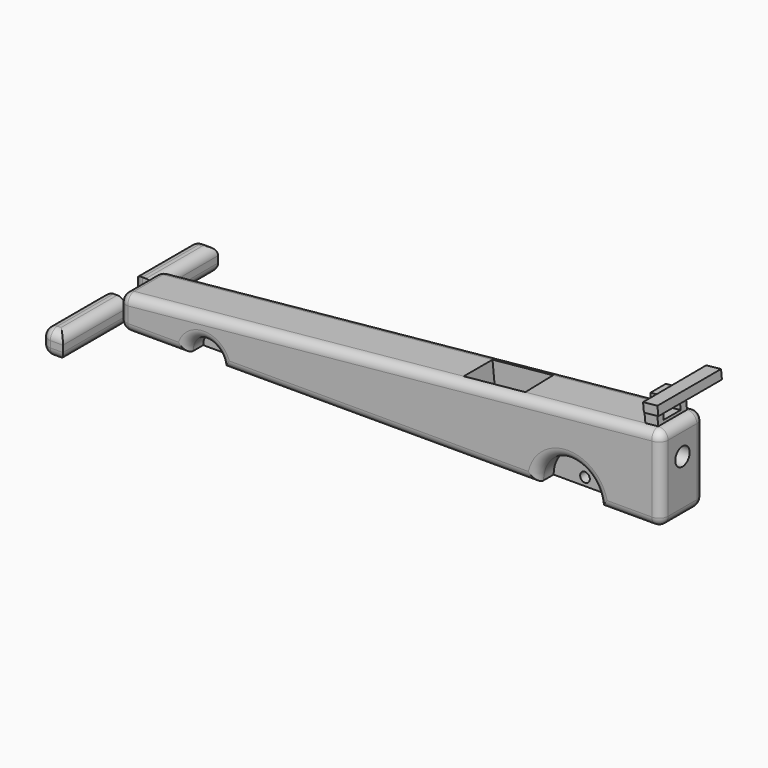
from build123d import *

# Parameters (mm, degrees)
F1_DEPTH        = 30
F2_R            = 10
F2_R_2          = 17.5
F3_DEPTH        = 12
F4_R            = 10
F4_R_2          = 17.5
F5_DEPTH        = 12
F6_R            = 5
F7_W            = 7.1860023443
F7_H            = 20
F8_DEPTH        = 10
F10_DEPTH       = 2.5
F12_DEPTH       = 5
F13_W           = 11.7590613663
F13_H           = 5.7444307604
F14_DEPTH       = 25
F15_R           = 2.0212258773
F16_DEPTH       = 25
F17_R           = 2.6949669584
F18_DEPTH       = 25
F19_W           = 44
F19_H           = 13.599084351
F20_DEPTH       = 12
F21_T1_DEPTH    = 20
F21_S5_W        = 5
F21_S5_H        = 5
F21_T6_DEPTH    = 5
F21_S11_W       = 5
F21_S11_H       = 5
F21_T12_DEPTH   = 5
F21_2_T1_DEPTH  = 51.5
F21_2_T3_DEPTH  = 34
F21_2_T5_DEPTH  = 3.599084351
F21_2_T7_DEPTH  = 21.099084351
F21_2_T9_DEPTH  = 19.5
F21_2_T11_DEPTH = 69
F21_2_S15_W     = 5
F21_2_S15_H     = 5
F21_2_T16_DEPTH = 5
F21_2_S21_W     = 5
F21_2_S21_H     = 5
F21_2_T22_DEPTH = 5
F21_2_S27_W     = 5
F21_2_S27_H     = 5
F21_2_T28_DEPTH = 5
F21_3_T1_DEPTH  = 51.5
F21_3_T3_DEPTH  = 3.5990095853
F21_3_T5_DEPTH  = 34.0000000001
F21_3_T7_DEPTH  = 19.4999760367
F21_3_T9_DEPTH  = 19.5
F21_3_T11_DEPTH = 21.0990747656
F21_3_T13_DEPTH = 69.0000000001
F21_3_T15_DEPTH = 19.5000239634
F21_3_T17_DEPTH = 69
F21_3_S21_W     = 5
F21_3_S21_H     = 5
F21_3_T22_DEPTH = 5
F21_3_T28_DEPTH = 5
F21_3_T34_DEPTH = 5
F23_DEPTH       = 15
F24_R           = 5
F25_DEPTH       = 10


# Not quite as in the source:
# - a fillet or chamfer that OpenCascade refuses, or shapes differently, is made with other operations: its cross-section is extruded or revolved along the edge and cut away or added


with BuildPart() as f1:
    # F0 (on Front) → F1 (new body)
    with BuildSketch(Plane.XZ):
        Polygon((-158.1492722034, -17.9878585041), (-158.1492722034, -36.1196212471), (143.4711813927, -36.1196212471), (143.4711813927, 11.656133458), align=None)
    extrude(amount=F1_DEPTH)

    # F2 (on face) → F3 (cut)
    with BuildSketch(Plane.XZ.offset(30)):
        with Locations((-110.8754724264, -36.1196212471)):
            Circle(F2_R)
        with Locations((91.665007174, -36.1196212471)):
            Circle(F2_R_2)
    extrude(amount=-F3_DEPTH, mode=Mode.SUBTRACT)

    # F4 (on face) → F5 (cut)
    with BuildSketch(Plane(origin=(0, 0, 0), x_dir=(-1, 0, 0), z_dir=(0, 1, 0))):
        with Locations((109.850294888, -36.1196212471)):
            Circle(F4_R)
        with Locations((-90.4239937663, -36.1196212471)):
            Circle(F4_R_2)
    extrude(amount=-F5_DEPTH, mode=Mode.SUBTRACT)

    # F6
    f6_edges = [f1.edges().sort_by_distance(p)[0] for p in [
        (-158.149272, -15, -17.987859),
        (-7.339045, -30, -3.165863),
        (-110.875472, -30, -26.119621),
        (-158.149272, -30, -27.05374),
        (91.665007, -30, -18.619621),
        (-158.149272, 0, -27.05374),
        (-109.850295, 0, -26.119621),
        (90.423994, 0, -18.619621),
        (-7.339045, 0, -3.165863),
        (143.471181, 0, -12.231744),
        (143.471181, -30, -12.231744),
        (143.471181, -15, 11.656133),
        (-13.463151, 0, -36.119621),
        (-13.355233, -30, -36.119621),
        (126.318094, -30, -36.119621),
        (125.697588, 0, -36.119621),
        (-138.999784, 0, -36.119621),
        (-139.512372, -30, -36.119621),
        (143.471181, -15, -36.119621),
    ]]
    fillet(f6_edges, radius=F6_R)

    # F7 (on face) → F8 (join)
    with BuildSketch(Plane(origin=(0.2379590763, 0, -2.4211760892), x_dir=(0.9952049917, 0, 0.0978111677), z_dir=(-0.0978111677, 0, 0.9952049917))):
        with Locations((134.814832017, -15)):
            Rectangle(F7_W, F7_H)
    extrude(amount=F8_DEPTH)

    # F9 (on face) → F10 (join)
    with BuildSketch(Plane(origin=(-0.7401526009, 0, 7.5308738276), x_dir=(0.9952049917, 0, 0.0978111677), z_dir=(-0.0978111677, 0, 0.9952049917))):
        Polygon((145.5644071102, -9.13162902), (131.2218308449, -9.2158466578), (131.2218308449, -19.9957098812), (145.5644071102, -19.9957098812), align=None)
    extrude(amount=F10_DEPTH)

    # F11 (on face) → F12 (join)
    with BuildSketch(Plane(origin=(-0.9846805202, 0, 10.0188863068), x_dir=(0.9952049917, 0, 0.0978111677), z_dir=(-0.0978111677, 0, 0.9952049917))):
        Polygon((150.0439193667, 6.3689760585), (141.7933106422, 6.3205296174), (142.0532540115, -37.9487908802), (150.0439193667, -37.8912001254), align=None)
    extrude(amount=F12_DEPTH)

    # F13 (on face) → F14 (cut)
    with BuildSketch(Plane(origin=(130.5926210745, 0, 12.8349605051), x_dir=(0, -1, 0), z_dir=(-0.9952049917, 0, -0.0978111677))):
        with Locations((15.0953773409, 1.9727416511)):
            Rectangle(F13_W, F13_H)
    extrude(amount=-F14_DEPTH, mode=Mode.SUBTRACT)

    # F15 (on face) → F16 (cut)
    with BuildSketch(Plane.XZ.offset(18)):
        with Locations((-111.3435998559, -32.4539355934)):
            Circle(F15_R)
    extrude(amount=-F16_DEPTH, mode=Mode.SUBTRACT)

    # F17 (on face) → F18 (cut)
    with BuildSketch(Plane.XZ.offset(18)):
        with Locations((91.6058570147, -31.7393243313)):
            Circle(F17_R)
    extrude(amount=-F18_DEPTH, mode=Mode.SUBTRACT)

    # F21: fillet of radius 5 on 1 edges, made by hand

    # F21_s2 → F21_t1 (cut)
    with BuildSketch(Plane.XZ.offset(5)):
        with BuildLine():
            ThreePointArc((-158.1492722034, -31.1196212471), (-156.6848061094, -34.655155153), (-153.1492722034, -36.1196212471))
            Line((-153.1492722034, -36.1196212471), (-158.1492722034, -36.1196212471))
            Line((-158.1492722034, -36.1196212471), (-158.1492722034, -31.1196212471))
        make_face()
    extrude(amount=F21_T1_DEPTH, mode=Mode.SUBTRACT)


with BuildPart() as f20:
    # F19 (on face) → F20 (new body)
    with BuildSketch(Plane(origin=(-158.1492722034, 0, 0), x_dir=(0, -1, 0), z_dir=(-1, 0, 0))):
        with Locations((-17, -29.3200790716)):
            Rectangle(F19_W, F19_H)
    extrude(amount=F20_DEPTH)

    # F21#2: fillet of radius 5 on 9 edges, made by hand

    # F21_2_s2 → F21_2_t1 (cut)
    with BuildSketch(Plane.XZ.offset(-34)):
        with BuildLine():
            ThreePointArc((-165.1492722034, -22.5205368961), (-168.6848061094, -23.9850029901), (-170.1492722034, -27.5205368961))
            Line((-170.1492722034, -27.5205368961), (-170.1492722034, -22.5205368961))
            Line((-170.1492722034, -22.5205368961), (-165.1492722034, -22.5205368961))
        make_face()
    extrude(amount=F21_2_T1_DEPTH, mode=Mode.SUBTRACT)

    # F21_2_s4 → F21_2_t3 (cut)
    with BuildSketch(Plane.XZ.offset(-34)):
        with BuildLine():
            ThreePointArc((-165.1492722034, -36.1196212471), (-168.6848061094, -34.655155153), (-170.1492722034, -31.1196212471))
            Line((-170.1492722034, -31.1196212471), (-170.1492722034, -36.1196212471))
            Line((-170.1492722034, -36.1196212471), (-165.1492722034, -36.1196212471))
        make_face()
    extrude(amount=F21_2_T3_DEPTH, mode=Mode.SUBTRACT)

    # F21_2_s6 → F21_2_t5 (cut)
    with BuildSketch(Plane.XY.offset(-31.1196212471)):
        with BuildLine():
            ThreePointArc((-165.1492722034, 39), (-168.6848061094, 37.5355339059), (-170.1492722034, 34))
            Line((-170.1492722034, 34), (-170.1492722034, 39))
            Line((-170.1492722034, 39), (-165.1492722034, 39))
        make_face()
    extrude(amount=F21_2_T5_DEPTH, mode=Mode.SUBTRACT)

    # F21_2_s8 → F21_2_t7 (cut)
    with BuildSketch(Plane.XY.offset(-31.1196212471)):
        with BuildLine():
            ThreePointArc((-165.1492722034, -5), (-168.6848061094, -3.5355339059), (-170.1492722034, 0))
            Line((-170.1492722034, 0), (-170.1492722034, -5))
            Line((-170.1492722034, -5), (-165.1492722034, -5))
        make_face()
    extrude(amount=F21_2_T7_DEPTH, mode=Mode.SUBTRACT)

    # F21_2_s10 → F21_2_t9 (cut)
    with BuildSketch(Plane.YZ.offset(-165.1492722034)):
        with BuildLine():
            ThreePointArc((34, -22.5205368961), (37.5355339059, -23.9850029901), (39, -27.5205368961))
            Line((39, -27.5205368961), (39, -22.5205368961))
            Line((39, -22.5205368961), (34, -22.5205368961))
        make_face()
        with BuildLine():
            ThreePointArc((39, -31.1196212471), (37.5355339059, -34.655155153), (34, -36.1196212471))
            Line((34, -36.1196212471), (39, -36.1196212471))
            Line((39, -36.1196212471), (39, -31.1196212471))
        make_face()
        with BuildLine():
            ThreePointArc((-5, -31.1196212471), (-3.5355339059, -34.655155153), (0, -36.1196212471))
            Line((0, -36.1196212471), (-5, -36.1196212471))
            Line((-5, -36.1196212471), (-5, -31.1196212471))
        make_face()
    extrude(amount=F21_2_T9_DEPTH, mode=Mode.SUBTRACT)

    # F21_2_s12 → F21_2_t11 (cut)
    with BuildSketch(Plane.XZ.offset(-51.5)):
        with BuildLine():
            ThreePointArc((-163.1492722034, -36.1196212471), (-159.6137382975, -34.655155153), (-158.1492722034, -31.1196212471))
            Line((-158.1492722034, -31.1196212471), (-158.1492722034, -36.1196212471))
            Line((-158.1492722034, -36.1196212471), (-163.1492722034, -36.1196212471))
        make_face()
        with BuildLine():
            ThreePointArc((-163.1492722034, -22.5205368961), (-159.6137382975, -23.9850029901), (-158.1492722034, -27.5205368961))
            Line((-158.1492722034, -27.5205368961), (-158.1492722034, -22.5205368961))
            Line((-158.1492722034, -22.5205368961), (-163.1492722034, -22.5205368961))
        make_face()
    extrude(amount=F21_2_T11_DEPTH, mode=Mode.SUBTRACT)


with BuildPart() as f20b:
    # F19 (on face) → F20, piece 2 (new body)
    with BuildSketch(Plane(origin=(-158.1492722034, 0, 0), x_dir=(0, -1, 0), z_dir=(-1, 0, 0))):
        Polygon((69, -22.5205368961), (25, -22.5205368961), (25, -36.1196212471), (69, -36.1195368961), align=None)
    extrude(amount=F20_DEPTH)

    # F21#3: fillet of radius 5 on 9 edges, made by hand

    # F21_3_s2 → F21_3_t1 (cut)
    with BuildSketch(Plane.XZ.offset(12.5)):
        with BuildLine():
            ThreePointArc((-165.1492722034, -22.5205368961), (-168.6848061094, -23.9850029901), (-170.1492722034, -27.5205368961))
            Line((-170.1492722034, -27.5205368961), (-170.1492722034, -22.5205368961))
            Line((-170.1492722034, -22.5205368961), (-165.1492722034, -22.5205368961))
        make_face()
    extrude(amount=F21_3_T1_DEPTH, mode=Mode.SUBTRACT)

    # F21_3_s4 → F21_3_t3 (cut)
    with BuildSketch(Plane.XY.offset(-31.1195464814)):
        with BuildLine():
            ThreePointArc((-165.1492722034, -69), (-168.6848061094, -67.5355339059), (-170.1492722034, -64))
            Line((-170.1492722034, -64), (-170.1492722034, -69))
            Line((-170.1492722034, -69), (-165.1492722034, -69))
        make_face()
    extrude(amount=F21_3_T3_DEPTH, mode=Mode.SUBTRACT)

    # F21_3_s6 → F21_3_t5 (cut)
    with BuildSketch(Plane(origin=(0, -29.9999403415, 5.75119e-05), x_dir=(1, 0, 0), z_dir=(0, -1, 1.9171e-06))):
        with BuildLine():
            ThreePointArc((-165.1492722034, -36.1196691737), (-168.6848061094, -34.6552030796), (-170.1492722034, -31.1196691737))
            Line((-170.1492722034, -31.1196691737), (-170.1492722034, -36.1196691737))
            Line((-170.1492722034, -36.1196691737), (-165.1492722034, -36.1196691737))
        make_face()
    extrude(amount=F21_3_T5_DEPTH, mode=Mode.SUBTRACT)

    # F21_3_s8 → F21_3_t7 (cut)
    with BuildSketch(Plane.YZ.offset(-165.1492722034)):
        with BuildLine():
            ThreePointArc((-69, -31.1195464814), (-67.5355372949, -34.6550769984), (-64.0000095853, -36.1195464814))
            Line((-64.0000095853, -36.1195464814), (-69, -36.1195368961))
            Line((-69, -36.1195368961), (-69, -31.1195464814))
        make_face()
    extrude(amount=F21_3_T7_DEPTH, mode=Mode.SUBTRACT)

    # F21_3_s10 → F21_3_t9 (cut)
    with BuildSketch(Plane.YZ.offset(-165.1492722034)):
        with BuildLine():
            ThreePointArc((-69, -27.5205368961), (-67.5355339059, -23.9850029901), (-64, -22.5205368961))
            Line((-64, -22.5205368961), (-69, -22.5205368961))
            Line((-69, -22.5205368961), (-69, -27.5205368961))
        make_face()
    extrude(amount=F21_3_T9_DEPTH, mode=Mode.SUBTRACT)

    # F21_3_s12 → F21_3_t11 (cut)
    with BuildSketch(Plane.XY.offset(-31.1196116617)):
        with BuildLine():
            ThreePointArc((-165.1492722034, -25), (-168.6848061094, -26.4644660941), (-170.1492722034, -30))
            Line((-170.1492722034, -30), (-170.1492722034, -25))
            Line((-170.1492722034, -25), (-165.1492722034, -25))
        make_face()
    extrude(amount=F21_3_T11_DEPTH, mode=Mode.SUBTRACT)

    # F21_3_s14 → F21_3_t13 (cut)
    with BuildSketch(Plane(origin=(0, -12.4999307562, 2.39632e-05), x_dir=(1, 0, 0), z_dir=(0, -1, 1.9171e-06))):
        with BuildLine():
            ThreePointArc((-163.1492722034, -36.1196691737), (-159.6137382975, -34.6552030796), (-158.1492722034, -31.1196691737))
            Line((-158.1492722034, -31.1196691737), (-158.1492722034, -36.1196691737))
            Line((-158.1492722034, -36.1196691737), (-163.1492722034, -36.1196691737))
        make_face()
    extrude(amount=F21_3_T13_DEPTH, mode=Mode.SUBTRACT)

    # F21_3_s16 → F21_3_t15 (cut)
    with BuildSketch(Plane.YZ.offset(-165.1492722034)):
        with BuildLine():
            ThreePointArc((-25, -31.1196116617), (-26.464469483, -34.6551489566), (-30.0000095853, -36.1196116617))
            Line((-30.0000095853, -36.1196116617), (-25, -36.1196212471))
            Line((-25, -36.1196212471), (-25, -31.1196116617))
        make_face()
    extrude(amount=F21_3_T15_DEPTH, mode=Mode.SUBTRACT)

    # F21_3_s18 → F21_3_t17 (cut)
    with BuildSketch(Plane.XZ.offset(12.5)):
        with BuildLine():
            ThreePointArc((-163.1492722034, -22.5205368961), (-159.6137382975, -23.9850029901), (-158.1492722034, -27.5205368961))
            Line((-158.1492722034, -27.5205368961), (-158.1492722034, -22.5205368961))
            Line((-158.1492722034, -22.5205368961), (-163.1492722034, -22.5205368961))
        make_face()
    extrude(amount=F21_3_T17_DEPTH, mode=Mode.SUBTRACT)


with BuildPart() as f21_tool4:
    # F21_s5 → F21_t6 (new body)
    with BuildSketch(Plane.YZ.offset(-153.1492722034)):
        with Locations((-2.5, -33.6196212471)):
            Rectangle(F21_S5_W, F21_S5_H)
    extrude(amount=-F21_T6_DEPTH)

    # F21_s7 → F21_t8 (revolve, cut)
    with BuildSketch(Plane(origin=(-153.1492722034, -5, -31.1196212471), x_dir=(0, -0.7071067812, 0.7071067812), z_dir=(0, -0.7071067812, -0.7071067812))):
        with BuildLine():
            ThreePointArc((0, -5), (5, 0), (0, 5))
            Line((0, 5), (0, -5))
        make_face()
    revolve(axis=Axis((-153.1492722034, -5, -31.1196212471), (-1, 0, 0)), mode=Mode.SUBTRACT)


with BuildPart() as f1_1:
    add(f1.part)

    # F21_t3: cut F21_tool4
    add(f21_tool4.part, mode=Mode.SUBTRACT)


with BuildPart() as f21_tool10:
    # F21_s11 → F21_t12 (new body)
    with BuildSketch(Plane.YZ.offset(-153.1492722034)):
        with Locations((-27.5, -33.6196212471)):
            Rectangle(F21_S11_W, F21_S11_H)
    extrude(amount=-F21_T12_DEPTH)

    # F21_s13 → F21_t14 (revolve, cut)
    with BuildSketch(Plane(origin=(-153.1492722034, -25, -31.1196212471), x_dir=(0, 0.7071067812, 0.7071067812), z_dir=(0, -0.7071067812, 0.7071067812))):
        with BuildLine():
            ThreePointArc((0, -5), (5, 0), (0, 5))
            Line((0, 5), (0, -5))
        make_face()
    revolve(axis=Axis((-153.1492722034, -25, -31.1196212471), (-1, 0, 0)), mode=Mode.SUBTRACT)


with BuildPart() as f1_2:
    add(f1_1.part)

    # F21_t9: cut F21_tool10
    add(f21_tool10.part, mode=Mode.SUBTRACT)

    # F22 (on face) → F23 (cut)
    with BuildSketch(Plane(origin=(0.2379590763, 0, -2.4211760892), x_dir=(0.9952049917, 0, 0.0978111677), z_dir=(-0.0978111677, 0, 0.9952049917))):
        Polygon((64.090423286, -25), (63.5211393237, -5), (29.6491980553, -5), (29.6491980553, -25), align=None)
    extrude(amount=-F23_DEPTH, mode=Mode.SUBTRACT)

    # F24 (on face) → F25 (cut)
    with BuildSketch(Plane.YZ.offset(143.4711813927)):
        with Locations((-15, -5.9098936617)):
            Circle(F24_R)
    extrude(amount=-F25_DEPTH, mode=Mode.SUBTRACT)


with BuildPart() as f21_2_tool14:
    # F21_2_s15 → F21_2_t16 (new body)
    with BuildSketch(Plane.XY.offset(-27.5205368961)):
        with Locations((-167.6492722034, 36.5)):
            Rectangle(F21_2_S15_W, F21_2_S15_H)
    extrude(amount=F21_2_T16_DEPTH)

    # F21_2_s17 → F21_2_t18 (revolve, cut)
    with BuildSketch(Plane(origin=(-165.1492722034, 34, -27.5205368961), x_dir=(0.7071067812, -0.7071067812, 0), z_dir=(-0.7071067812, -0.7071067812, 0))):
        with BuildLine():
            ThreePointArc((0, -5), (5, 0), (0, 5))
            Line((0, 5), (0, -5))
        make_face()
    revolve(axis=Axis((-165.1492722034, 34, -27.5205368961), (0, 0, 1)), mode=Mode.SUBTRACT)


with BuildPart() as f20_1:
    add(f20.part)

    # F21_2_t13: cut F21_2_tool14
    add(f21_2_tool14.part, mode=Mode.SUBTRACT)


with BuildPart() as f21_2_tool20:
    # F21_2_s21 → F21_2_t22 (new body)
    with BuildSketch(Plane.XZ.offset(-34)):
        with Locations((-167.6492722034, -33.6196212471)):
            Rectangle(F21_2_S21_W, F21_2_S21_H)
    extrude(amount=-F21_2_T22_DEPTH)

    # F21_2_s23 → F21_2_t24 (revolve, cut)
    with BuildSketch(Plane(origin=(-165.1492722034, 34, -31.1196212471), x_dir=(0.7071067812, 0, 0.7071067812), z_dir=(-0.7071067812, 0, 0.7071067812))):
        with BuildLine():
            ThreePointArc((0, -5), (5, 0), (0, 5))
            Line((0, 5), (0, -5))
        make_face()
    revolve(axis=Axis((-165.1492722034, 34, -31.1196212471), (0, 1, 0)), mode=Mode.SUBTRACT)


with BuildPart() as f20_2:
    add(f20_1.part)

    # F21_2_t19: cut F21_2_tool20
    add(f21_2_tool20.part, mode=Mode.SUBTRACT)


with BuildPart() as f21_2_tool26:
    # F21_2_s27 → F21_2_t28 (new body)
    with BuildSketch(Plane.XZ):
        with Locations((-167.6492722034, -33.6196212471)):
            Rectangle(F21_2_S27_W, F21_2_S27_H)
    extrude(amount=F21_2_T28_DEPTH)

    # F21_2_s29 → F21_2_t30 (revolve, cut)
    with BuildSketch(Plane(origin=(-165.1492722034, 0, -31.1196212471), x_dir=(0.7071067812, 0, 0.7071067812), z_dir=(0.7071067812, 0, -0.7071067812))):
        with BuildLine():
            ThreePointArc((0, -5), (5, 0), (0, 5))
            Line((0, 5), (0, -5))
        make_face()
    revolve(axis=Axis((-165.1492722034, 0, -31.1196212471), (0, -1, 0)), mode=Mode.SUBTRACT)


with BuildPart() as f20_3:
    add(f20_2.part)

    # F21_2_t25: cut F21_2_tool26
    add(f21_2_tool26.part, mode=Mode.SUBTRACT)


with BuildPart() as f21_3_tool20:
    # F21_3_s21 → F21_3_t22 (new body)
    with BuildSketch(Plane.XZ.offset(64)):
        with Locations((-167.6492722034, -25.0205368961)):
            Rectangle(F21_3_S21_W, F21_3_S21_H)
    extrude(amount=F21_3_T22_DEPTH)

    # F21_3_s23 → F21_3_t24 (revolve, cut)
    with BuildSketch(Plane(origin=(-165.1492722034, -64, -27.5205368961), x_dir=(0.7071067812, 0, -0.7071067812), z_dir=(-0.7071067812, 0, -0.7071067812))):
        with BuildLine():
            ThreePointArc((0, -5), (5, 0), (0, 5))
            Line((0, 5), (0, -5))
        make_face()
    revolve(axis=Axis((-165.1492722034, -64, -27.5205368961), (0, -1, 0)), mode=Mode.SUBTRACT)


with BuildPart() as f20b_1:
    add(f20b.part)

    # F21_3_t19: cut F21_3_tool20
    add(f21_3_tool20.part, mode=Mode.SUBTRACT)


with BuildPart() as f21_3_tool26:
    # F21_3_s27 → F21_3_t28 (new body)
    with BuildSketch(Plane.YZ.offset(-165.1492722034)):
        Polygon((-64, -31.1195464814), (-69, -31.1195464814), (-69, -36.1195368961), (-64.0000095853, -36.1195464814), align=None)
    extrude(amount=-F21_3_T28_DEPTH)

    # F21_3_s29 → F21_3_t30 (revolve, cut)
    with BuildSketch(Plane(origin=(-165.1492722034, -64, -31.1195464814), x_dir=(0, 0.707107459, 0.7071061034), z_dir=(0, -0.7071061034, 0.707107459))):
        with BuildLine():
            ThreePointArc((0, -5), (5, 0), (0, 5))
            Line((0, 5), (0, -5))
        make_face()
    revolve(axis=Axis((-165.1492722034, -64, -31.1195464814), (-1, 0, 0)), mode=Mode.SUBTRACT)


with BuildPart() as f20b_2:
    add(f20b_1.part)

    # F21_3_t25: cut F21_3_tool26
    add(f21_3_tool26.part, mode=Mode.SUBTRACT)


with BuildPart() as f21_3_tool32:
    # F21_3_s33 → F21_3_t34 (new body)
    with BuildSketch(Plane.YZ.offset(-165.1492722034)):
        Polygon((-30, -31.1196116617), (-25, -31.1196116617), (-25, -36.1196212471), (-30.0000095853, -36.1196116617), align=None)
    extrude(amount=-F21_3_T34_DEPTH)

    # F21_3_s35 → F21_3_t36 (revolve, cut)
    with BuildSketch(Plane(origin=(-165.1492722034, -30, -31.1196116617), x_dir=(0, -0.7071061034, 0.707107459), z_dir=(0, -0.707107459, -0.7071061034))):
        with BuildLine():
            ThreePointArc((0, -5), (5, 0), (0, 5))
            Line((0, 5), (0, -5))
        make_face()
    revolve(axis=Axis((-165.1492722034, -30, -31.1196116617), (-1, 0, 0)), mode=Mode.SUBTRACT)


with BuildPart() as f20b_3:
    add(f20b_2.part)

    # F21_3_t31: cut F21_3_tool32
    add(f21_3_tool32.part, mode=Mode.SUBTRACT)


solid = Compound([f1_2.part, f20_3.part, f20b_3.part])
